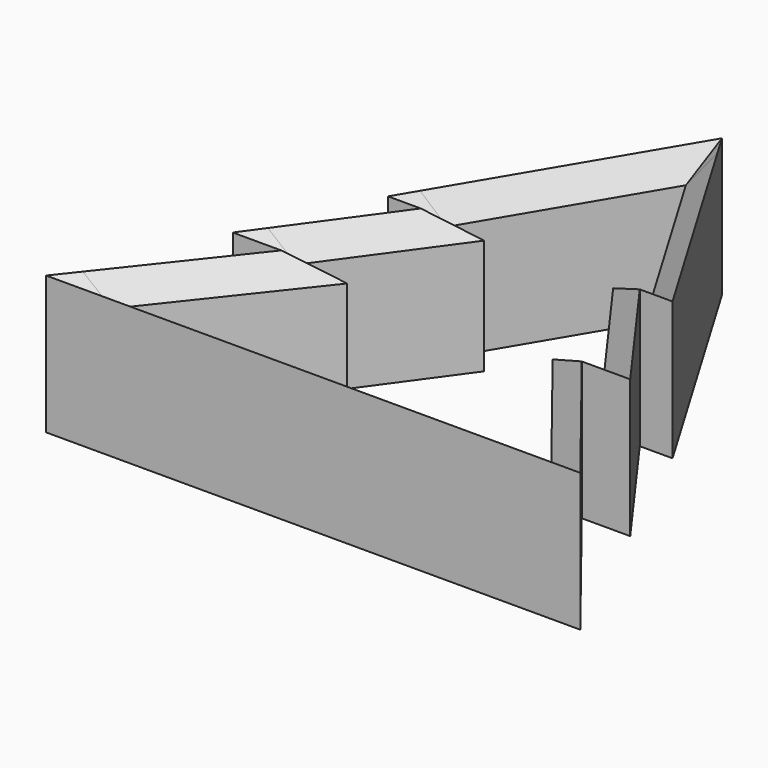
from build123d import *

# Parameters (mm, degrees)
F1_DEPTH     = 25.4
F2_T4_DEPTH  = 57.8731292872
F2_T9_DEPTH  = 41.0926802964
F2_T14_DEPTH = 63.860720941
F2_T19_DEPTH = 105.3637727113
F2_T25_DEPTH = 63.860720941
F2_T30_DEPTH = 41.0926802964
F2_T35_DEPTH = 57.8731292872
F2_T40_DEPTH = 38.84406527
F2_T45_DEPTH = 65.6766537471
F2_T51_DEPTH = 65.6766537471
F2_T57_DEPTH = 38.84406527


# Not quite as in the source:
# - a fillet or chamfer that OpenCascade refuses, or shapes differently, is made with other operations: its cross-section is extruded or revolved along the edge and cut away or added


with BuildPart() as f1:
    # F0 (on Top) → F1 (new body)
    with BuildSketch(Plane.XY):
        Polygon((-44.2180235174, 0.5666213692), (0, 0.5666213692), (44.2180235174, 0.5666213692), (24.8746419192, 25.0471287349), (32.8946120205, 25.0471287349), (18.1270946377, 45.4824770849), (23.5501605907, 45.4824770849), (0, 85.1436531389), (-23.5501605907, 45.4824770849), (-18.1270946377, 45.4824770849), (-32.8946120205, 25.0471287349), (-24.8746419192, 25.0471287349), align=None)
        Polygon((36.3516993821, 4.3766213692), (0, 4.3766213692), (-36.3516993821, 4.3766213692), (-17.0083177839, 28.8571287349), (-25.4406241332, 28.8571287349), (-10.6731067504, 49.2924770849), (-16.8567980732, 49.2924770849), (0, 77.6812616757), (16.8567980732, 49.2924770849), (10.6731067504, 49.2924770849), (25.4406241332, 28.8571287349), (17.0083177839, 28.8571287349), align=None, mode=Mode.SUBTRACT)
    extrude(amount=F1_DEPTH)

    # F2: chamfer of 6.35 on 11 edges, made by hand


with BuildPart() as f2_tool2:
    # F2_s3 → F2_t4 (new body)
    with BuildSketch(Plane(origin=(-29.3040400955, 40.5510453716, 0), x_dir=(0, 0, 1), z_dir=(0.585716126, -0.8105162674, 0))):
        Polygon((25.4, -43.8721253629), (19.05, -37.5221253629), (25.4, -37.5221253629), align=None)
    extrude(amount=F2_T4_DEPTH)

    split(bisect_by=Plane(origin=(0, 23.9535643674, 23.9535643674), x_dir=(1, 0, 0), z_dir=(0, 0.7071067812, 0.7071067812)), keep=Keep.TOP)


with BuildPart() as f1_1:
    add(f1.part)

    # F2_t1: cut F2_tool2
    add(f2_tool2.part, mode=Mode.SUBTRACT)


with BuildPart() as f2_tool7:
    # F2_s8 → F2_t9 (new body)
    with BuildSketch(Plane.YZ.offset(41.7708111067)):
        Polygon((22.5071287349, 25.4), (28.8571287349, 19.05), (28.8571287349, 25.4), align=None)
    extrude(amount=-F2_T9_DEPTH)

    split(bisect_by=Plane(origin=(7.4859790504, 5.409710853, -9.2360626814), x_dir=(0.585716126, -0.8105162674, 0), z_dir=(-0.573121549, -0.4141638445, 0.7071067812)), keep=Keep.TOP)


with BuildPart() as f1_2:
    add(f1_1.part)

    # F2_t6: cut F2_tool7
    add(f2_tool7.part, mode=Mode.SUBTRACT)


with BuildPart() as f2_tool12:
    # F2_s13 → F2_t14 (new body)
    with BuildSketch(Plane(origin=(-17.6242588903, 22.3048280047, 0), x_dir=(0, 0, 1), z_dir=(0.6199732843, -0.7846229201, 0))):
        Polygon((25.4, -37.5857648435), (19.05, -31.2357648435), (25.4, -31.2357648435), align=None)
    extrude(amount=F2_T14_DEPTH)

    split(bisect_by=Plane(origin=(0, 11.7133106846, 11.7133106846), x_dir=(1, 0, 0), z_dir=(0, 0.7071067812, 0.7071067812)), keep=Keep.TOP)


with BuildPart() as f1_3:
    add(f1_2.part)

    # F2_t11: cut F2_tool12
    add(f2_tool12.part, mode=Mode.SUBTRACT)


with BuildPart() as f2_tool17:
    # F2_s18 → F2_t19 (new body)
    with BuildSketch(Plane.YZ.offset(-52.6818863557)):
        Polygon((-1.9733786308, 25.4), (4.3766213692, 19.05), (4.3766213692, 25.4), align=None)
    extrude(amount=F2_T19_DEPTH)

    split(bisect_by=Plane(origin=(4.7806151974, 3.7774243261, -6.0928824217), x_dir=(0.6199732843, -0.7846229201, 0), z_dir=(-0.5548121875, -0.4383873135, 0.7071067812)), keep=Keep.TOP)

    split(bisect_by=Plane(origin=(-4.7806151974, 3.7774243261, -6.0928824217), x_dir=(0.6199732843, 0.7846229201, 0), z_dir=(0.5548121875, -0.4383873135, 0.7071067812)), keep=Keep.TOP)


with BuildPart() as f1_4:
    add(f1_3.part)

    # F2_t16: cut F2_tool17
    add(f2_tool17.part, mode=Mode.SUBTRACT)


with BuildPart() as f2_tool23:
    # F2_s24 → F2_t25 (new body)
    with BuildSketch(Plane(origin=(-21.9676820116, -27.8017573382, 0), x_dir=(0, 0, 1), z_dir=(0.6199732843, 0.7846229201, 0))):
        Polygon((25.4, -37.5857648435), (19.05, -31.2357648435), (25.4, -31.2357648435), align=None)
    extrude(amount=F2_T25_DEPTH)

    split(bisect_by=Plane(origin=(0, 11.7133106846, 11.7133106846), x_dir=(1, 0, 0), z_dir=(0, 0.7071067812, 0.7071067812)), keep=Keep.TOP)


with BuildPart() as f1_5:
    add(f1_4.part)

    # F2_t22: cut F2_tool23
    add(f2_tool23.part, mode=Mode.SUBTRACT)


with BuildPart() as f2_tool28:
    # F2_s29 → F2_t30 (new body)
    with BuildSketch(Plane.YZ.offset(-0.6781308103)):
        Polygon((22.5071287349, 25.4), (28.8571287349, 19.05), (28.8571287349, 25.4), align=None)
    extrude(amount=-F2_T30_DEPTH)

    split(bisect_by=Plane(origin=(-7.4859790504, 5.409710853, -9.2360626814), x_dir=(0.585716126, 0.8105162674, 0), z_dir=(0.573121549, -0.4141638445, 0.7071067812)), keep=Keep.TOP)


with BuildPart() as f1_6:
    add(f1_5.part)

    # F2_t27: cut F2_tool28
    add(f2_tool28.part, mode=Mode.SUBTRACT)


with BuildPart() as f2_tool33:
    # F2_s34 → F2_t35 (new body)
    with BuildSketch(Plane(origin=(-4.5931849883, -6.3560673631, 0), x_dir=(0, 0, 1), z_dir=(0.585716126, 0.8105162674, 0))):
        Polygon((25.4, -43.8721253629), (19.05, -37.5221253629), (25.4, -37.5221253629), align=None)
    extrude(amount=F2_T35_DEPTH)

    split(bisect_by=Plane(origin=(0, 23.9535643674, 23.9535643674), x_dir=(1, 0, 0), z_dir=(0, 0.7071067812, 0.7071067812)), keep=Keep.TOP)


with BuildPart() as f1_7:
    add(f1_6.part)

    # F2_t32: cut F2_tool33
    add(f2_tool33.part, mode=Mode.SUBTRACT)


with BuildPart() as f2_tool38:
    # F2_s39 → F2_t40 (new body)
    with BuildSketch(Plane.YZ.offset(5.6570802232)):
        Polygon((42.9424770849, 25.4), (49.2924770849, 19.05), (49.2924770849, 25.4), align=None)
    extrude(amount=-F2_T40_DEPTH)

    split(bisect_by=Plane(origin=(-8.8610845664, 5.2615677423, -10.3054798432), x_dir=(0.5105601896, 0.8598420162, 0), z_dir=(0.6080001204, -0.3610205722, 0.7071067812)), keep=Keep.TOP)


with BuildPart() as f1_8:
    add(f1_7.part)

    # F2_t37: cut F2_tool38
    add(f2_tool38.part, mode=Mode.SUBTRACT)


with BuildPart() as f2_tool43:
    # F2_s44 → F2_t45 (new body)
    with BuildSketch(Plane(origin=(8.9078181115, 15.0017890968, 0), x_dir=(0, 0, 1), z_dir=(0.5105601896, 0.8598420162, 0))):
        Polygon((25.4, -46.0109596864), (19.05, -39.6609596864), (25.4, -39.6609596864), align=None)
    extrude(amount=F2_T45_DEPTH)

    split(bisect_by=Plane(origin=(0, 34.1712385424, 34.1712385424), x_dir=(1, 0, 0), z_dir=(0, 0.7071067812, 0.7071067812)), keep=Keep.TOP)

    split(bisect_by=Plane(origin=(8.8610845664, 5.2615677423, -10.3054798432), x_dir=(0.5105601896, -0.8598420162, 0), z_dir=(-0.6080001204, -0.3610205722, 0.7071067812)), keep=Keep.TOP)


with BuildPart() as f1_9:
    add(f1_8.part)

    # F2_t42: cut F2_tool43
    add(f2_tool43.part, mode=Mode.SUBTRACT)


with BuildPart() as f2_tool49:
    # F2_s50 → F2_t51 (new body)
    with BuildSketch(Plane(origin=(-42.4397028983, 71.4733354725, 0), x_dir=(0, 0, 1), z_dir=(0.5105601896, -0.8598420162, 0))):
        Polygon((25.4, -46.0109596864), (19.05, -39.6609596864), (25.4, -39.6609596864), align=None)
    extrude(amount=F2_T51_DEPTH)

    split(bisect_by=Plane(origin=(-8.8610845664, 5.2615677423, -10.3054798432), x_dir=(0.5105601896, 0.8598420162, 0), z_dir=(0.6080001204, -0.3610205722, 0.7071067812)), keep=Keep.TOP)

    split(bisect_by=Plane(origin=(0, 34.1712385424, 34.1712385424), x_dir=(1, 0, 0), z_dir=(0, 0.7071067812, 0.7071067812)), keep=Keep.TOP)


with BuildPart() as f1_10:
    add(f1_9.part)

    # F2_t48: cut F2_tool49
    add(f2_tool49.part, mode=Mode.SUBTRACT)


with BuildPart() as f2_tool55:
    # F2_s56 → F2_t57 (new body)
    with BuildSketch(Plane.YZ.offset(33.1869850468)):
        Polygon((42.9424770849, 25.4), (49.2924770849, 19.05), (49.2924770849, 25.4), align=None)
    extrude(amount=-F2_T57_DEPTH)

    split(bisect_by=Plane(origin=(8.8610845664, 5.2615677423, -10.3054798432), x_dir=(0.5105601896, -0.8598420162, 0), z_dir=(-0.6080001204, -0.3610205722, 0.7071067812)), keep=Keep.TOP)


with BuildPart() as f1_11:
    add(f1_10.part)

    # F2_t54: cut F2_tool55
    add(f2_tool55.part, mode=Mode.SUBTRACT)


solid = f1_11.part
